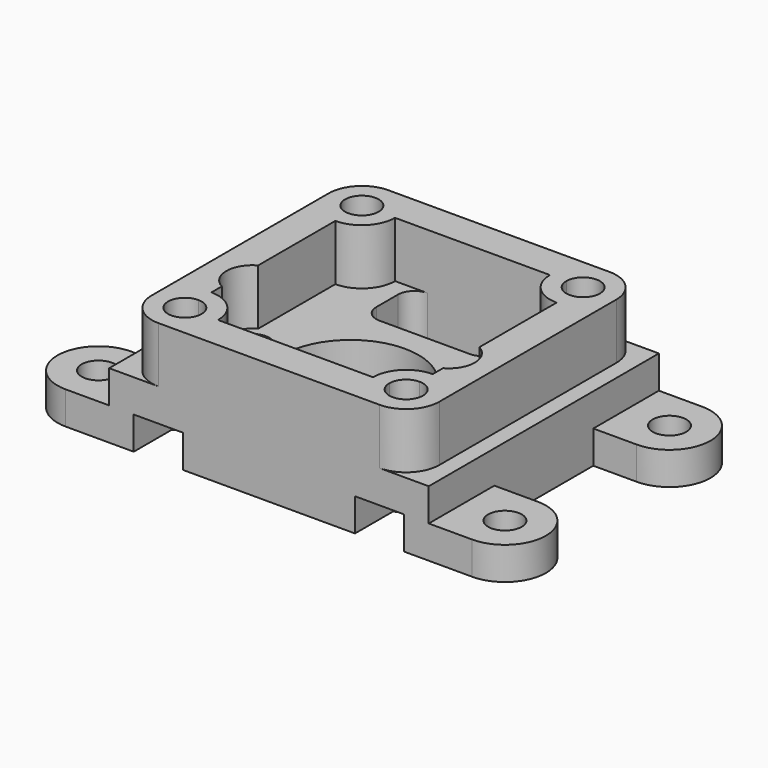
from build123d import *

# Parameters (mm, degrees)
F0_R     = 8.3
F1_DEPTH = 14.8
F0_R_2   = 2.05
F2_DEPTH = 4
F3_DEPTH = 4
F4_R     = 8.3
F5_DEPTH = 6.8
F6_DEPTH = 8


# Not quite as in the source:
# - a feature names something its author has since deleted; it is built from what else it names


with BuildPart() as f1:
    # F0 (on Top) → F1 (new body)
    with BuildSketch(Plane.XY):
        with BuildLine():
            Line((-16.5, 15.2320508076), (-16.5, 17.55))
            Line((-16.5, 17.55), (-17.55, 17.55))
            Line((-17.55, 17.55), (-19.5, 17.55))
            Line((-19.5, 17.55), (-19.5, 7.55))
            Line((-19.5, 7.55), (-19.5, -7.55))
            Line((-19.5, -7.55), (-19.5, -17.55))
            Line((-19.5, -17.55), (-17.55, -17.55))
            Line((-17.55, -17.55), (-16.5, -17.55))
            Line((-16.5, -17.55), (-16.5, -15.2320508076))
            Line((-16.5, -15.2320508076), (-16.5, -11.7679491924))
            Line((-16.5, -11.7679491924), (-13.5, -10.0358983849))
            Line((-13.5, -10.0358983849), (-13.5, -7.8699277969))
            ThreePointArc((-13.5, -7.8699277969), (-15.15, -5.1), (-13.5, -2.3300722031))
            Line((-13.5, -2.3300722031), (-13.5, 10.0358983849))
            Line((-13.5, 10.0358983849), (-16.5, 11.7679491924))
            Line((-16.5, 11.7679491924), (-16.5, 15.2320508076))
        make_face()
        with BuildLine():
            Line((10.5, 11.7679491924), (10.5, 13.5))
            Line((10.5, 13.5), (5.5, 13.5))
            ThreePointArc((5.5, 13.5), (6.9142135624, 12.9142135624), (7.5, 11.5))
            Line((7.5, 11.5), (7.5, 8.2))
            ThreePointArc((7.5, 8.2), (6.9142135624, 6.7857864376), (5.5, 6.2))
            Line((5.5, 6.2), (-5.5, 6.2))
            ThreePointArc((-5.5, 6.2), (-6.9142135624, 6.7857864376), (-7.5, 8.2))
            Line((-7.5, 8.2), (-7.5, 11.5))
            ThreePointArc((-7.5, 11.5), (-6.9142135624, 12.9142135624), (-5.5, 13.5))
            Line((-5.5, 13.5), (-10.5, 13.5))
            Line((-10.5, 13.5), (-10.5, 11.7679491924))
            Line((-10.5, 11.7679491924), (-13.5, 10.0358983849))
            Line((-13.5, 10.0358983849), (-13.5, -2.3300722031))
            ThreePointArc((-13.5, -2.3300722031), (-10.3879361055, -2.3937572171), (-8.85, -5.1))
            ThreePointArc((-8.85, -5.1), (-10.3879361055, -7.8062427829), (-13.5, -7.8699277969))
            Line((-13.5, -7.8699277969), (-13.5, -10.0358983849))
            Line((-13.5, -10.0358983849), (-10.5, -11.7679491924))
            Line((-10.5, -11.7679491924), (-10.5, -13.5))
            Line((-10.5, -13.5), (10.5, -13.5))
            Line((10.5, -13.5), (10.5, -11.7679491924))
            Line((10.5, -11.7679491924), (13.5, -10.0358983849))
            Line((13.5, -10.0358983849), (13.5, -7.8699277969))
            ThreePointArc((13.5, -7.8699277969), (8.85, -5.1), (13.5, -2.3300722031))
            Line((13.5, -2.3300722031), (13.5, 10.0358983849))
            Line((13.5, 10.0358983849), (10.5, 11.7679491924))
        make_face()
        with Locations((0, -5.1)):
            Circle(F0_R, mode=Mode.SUBTRACT)
        Polygon((10.5, 15.2320508076), (10.5, 17.55), (-10.5, 17.55), (-10.5, 15.2320508076), (-10.5, 13.5), (-5.5, 13.5), (5.5, 13.5), (10.5, 13.5), align=None)
        with BuildLine():
            Line((19.5, 17.55), (17.55, 17.55))
            Line((17.55, 17.55), (16.5, 17.55))
            Line((16.5, 17.55), (16.5, 15.2320508076))
            Line((16.5, 15.2320508076), (16.5, 11.7679491924))
            Line((16.5, 11.7679491924), (13.5, 10.0358983849))
            Line((13.5, 10.0358983849), (13.5, -2.3300722031))
            ThreePointArc((13.5, -2.3300722031), (14.7062427829, -3.4879361055), (15.15, -5.1))
            ThreePointArc((15.15, -5.1), (14.7062427829, -6.7120638945), (13.5, -7.8699277969))
            Line((13.5, -7.8699277969), (13.5, -10.0358983849))
            Line((13.5, -10.0358983849), (16.5, -11.7679491924))
            Line((16.5, -11.7679491924), (16.5, -15.2320508076))
            Line((16.5, -15.2320508076), (16.5, -17.55))
            Line((16.5, -17.55), (17.55, -17.55))
            Line((17.55, -17.55), (19.5, -17.55))
            Line((19.5, -17.55), (19.5, -7.55))
            Line((19.5, -7.55), (19.5, 7.55))
            Line((19.5, 7.55), (19.5, 17.55))
        make_face()
        Polygon((-10.5, -17.55), (10.5, -17.55), (10.5, -15.2320508076), (10.5, -13.5), (-10.5, -13.5), (-10.5, -15.2320508076), align=None)
        Polygon((-10.5, 15.2320508076), (-10.5, 17.55), (-16.5, 17.55), (-16.5, 15.2320508076), (-13.5, 16.9641016151), align=None)
        with BuildLine():
            Line((-10.5, 13.5), (-10.5, 15.2320508076))
            Line((-10.5, 15.2320508076), (-13.5, 16.9641016151))
            Line((-13.5, 16.9641016151), (-16.5, 15.2320508076))
            Line((-16.5, 15.2320508076), (-16.5, 11.7679491924))
            Line((-16.5, 11.7679491924), (-13.5, 10.0358983849))
            Line((-13.5, 10.0358983849), (-13.5, 11.45))
            ThreePointArc((-13.5, 11.45), (-14.9495689014, 14.9495689014), (-11.45, 13.5))
            Line((-11.45, 13.5), (-10.5, 13.5))
        make_face()
        Polygon((16.5, 15.2320508076), (16.5, 17.55), (10.5, 17.55), (10.5, 15.2320508076), (13.5, 16.9641016151), align=None)
        with BuildLine():
            Line((16.5, 11.7679491924), (16.5, 15.2320508076))
            Line((16.5, 15.2320508076), (13.5, 16.9641016151))
            Line((13.5, 16.9641016151), (10.5, 15.2320508076))
            Line((10.5, 15.2320508076), (10.5, 13.5))
            Line((10.5, 13.5), (11.45, 13.5))
            ThreePointArc((11.45, 13.5), (13.5, 15.55), (15.55, 13.5))
            ThreePointArc((15.55, 13.5), (14.9495689014, 12.0504310986), (13.5, 11.45))
            Line((13.5, 11.45), (13.5, 10.0358983849))
            Line((13.5, 10.0358983849), (16.5, 11.7679491924))
        make_face()
        with BuildLine():
            Line((11.45, 13.5), (10.5, 13.5))
            Line((10.5, 13.5), (10.5, 11.7679491924))
            Line((10.5, 11.7679491924), (13.5, 10.0358983849))
            Line((13.5, 10.0358983849), (13.5, 11.45))
            ThreePointArc((13.5, 11.45), (12.0504310986, 12.0504310986), (11.45, 13.5))
        make_face()
        with BuildLine():
            Line((-10.5, 11.7679491924), (-10.5, 13.5))
            Line((-10.5, 13.5), (-11.45, 13.5))
            ThreePointArc((-11.45, 13.5), (-12.0504310986, 12.0504310986), (-13.5, 11.45))
            Line((-13.5, 11.45), (-13.5, 10.0358983849))
            Line((-13.5, 10.0358983849), (-10.5, 11.7679491924))
        make_face()
        with BuildLine():
            Line((-10.5, -11.7679491924), (-13.5, -10.0358983849))
            Line((-13.5, -10.0358983849), (-13.5, -11.45))
            ThreePointArc((-13.5, -11.45), (-12.0504310986, -12.0504310986), (-11.45, -13.5))
            Line((-11.45, -13.5), (-10.5, -13.5))
            Line((-10.5, -13.5), (-10.5, -11.7679491924))
        make_face()
        with BuildLine():
            Line((-13.5, -16.9641016151), (-10.5, -15.2320508076))
            Line((-10.5, -15.2320508076), (-10.5, -13.5))
            Line((-10.5, -13.5), (-11.45, -13.5))
            ThreePointArc((-11.45, -13.5), (-14.9495689014, -14.9495689014), (-13.5, -11.45))
            Line((-13.5, -11.45), (-13.5, -10.0358983849))
            Line((-13.5, -10.0358983849), (-16.5, -11.7679491924))
            Line((-16.5, -11.7679491924), (-16.5, -15.2320508076))
            Line((-16.5, -15.2320508076), (-13.5, -16.9641016151))
        make_face()
        Polygon((-16.5, -17.55), (-10.5, -17.55), (-10.5, -15.2320508076), (-13.5, -16.9641016151), (-16.5, -15.2320508076), align=None)
        Polygon((10.5, -17.55), (16.5, -17.55), (16.5, -15.2320508076), (13.5, -16.9641016151), (10.5, -15.2320508076), align=None)
        with BuildLine():
            Line((16.5, -11.7679491924), (13.5, -10.0358983849))
            Line((13.5, -10.0358983849), (13.5, -11.45))
            ThreePointArc((13.5, -11.45), (14.9495689014, -12.0504310986), (15.55, -13.5))
            ThreePointArc((15.55, -13.5), (13.5, -15.55), (11.45, -13.5))
            Line((11.45, -13.5), (10.5, -13.5))
            Line((10.5, -13.5), (10.5, -15.2320508076))
            Line((10.5, -15.2320508076), (13.5, -16.9641016151))
            Line((13.5, -16.9641016151), (16.5, -15.2320508076))
            Line((16.5, -15.2320508076), (16.5, -11.7679491924))
        make_face()
        with BuildLine():
            Line((13.5, -11.45), (13.5, -10.0358983849))
            Line((13.5, -10.0358983849), (10.5, -11.7679491924))
            Line((10.5, -11.7679491924), (10.5, -13.5))
            Line((10.5, -13.5), (11.45, -13.5))
            ThreePointArc((11.45, -13.5), (12.0504310986, -12.0504310986), (13.5, -11.45))
        make_face()
    extrude(amount=F1_DEPTH)

    # F0 (on Top) → F2 (join)
    with BuildSketch(Plane.XY):
        with BuildLine():
            Line((-19.5, 7.55), (-19.5, 17.55))
            Line((-19.5, 17.55), (-24.8, 17.55))
            ThreePointArc((-24.8, 17.55), (-29.8, 12.55), (-24.8, 7.55))
            Line((-24.8, 7.55), (-19.5, 7.55))
        make_face()
        with Locations((-24.8, 12.55)):
            Circle(F0_R_2, mode=Mode.SUBTRACT)
        with BuildLine():
            Line((-19.5, -17.55), (-19.5, -7.55))
            Line((-19.5, -7.55), (-24.8, -7.55))
            ThreePointArc((-24.8, -7.55), (-29.8, -12.55), (-24.8, -17.55))
            Line((-24.8, -17.55), (-19.5, -17.55))
        make_face()
        with Locations((-24.8, -12.55)):
            Circle(F0_R_2, mode=Mode.SUBTRACT)
        with BuildLine():
            Line((24.8, -7.55), (19.5, -7.55))
            Line((19.5, -7.55), (19.5, -17.55))
            Line((19.5, -17.55), (24.8, -17.55))
            ThreePointArc((24.8, -17.55), (29.8, -12.55), (24.8, -7.55))
        make_face()
        with Locations((24.8, -12.55)):
            Circle(F0_R_2, mode=Mode.SUBTRACT)
        with BuildLine():
            Line((24.8, 17.55), (19.5, 17.55))
            Line((19.5, 17.55), (19.5, 7.55))
            Line((19.5, 7.55), (24.8, 7.55))
            ThreePointArc((24.8, 7.55), (29.8, 12.55), (24.8, 17.55))
        make_face()
        with Locations((24.8, 12.55)):
            Circle(F0_R_2, mode=Mode.SUBTRACT)
    extrude(amount=F2_DEPTH)

    # F0 (on Top) → F3 (cut)
    with BuildSketch(Plane.XY):
        with BuildLine():
            Line((16.5, 11.7679491924), (16.5, 15.2320508076))
            Line((16.5, 15.2320508076), (13.5, 16.9641016151))
            Line((13.5, 16.9641016151), (10.5, 15.2320508076))
            Line((10.5, 15.2320508076), (10.5, 13.5))
            Line((10.5, 13.5), (11.45, 13.5))
            ThreePointArc((11.45, 13.5), (13.5, 15.55), (15.55, 13.5))
            ThreePointArc((15.55, 13.5), (14.9495689014, 12.0504310986), (13.5, 11.45))
            Line((13.5, 11.45), (13.5, 10.0358983849))
            Line((13.5, 10.0358983849), (16.5, 11.7679491924))
        make_face()
        with BuildLine():
            Line((11.45, 13.5), (10.5, 13.5))
            Line((10.5, 13.5), (10.5, 11.7679491924))
            Line((10.5, 11.7679491924), (13.5, 10.0358983849))
            Line((13.5, 10.0358983849), (13.5, 11.45))
            ThreePointArc((13.5, 11.45), (12.0504310986, 12.0504310986), (11.45, 13.5))
        make_face()
        Polygon((16.5, 15.2320508076), (16.5, 17.55), (10.5, 17.55), (10.5, 15.2320508076), (13.5, 16.9641016151), align=None)
        with BuildLine():
            Line((-10.5, 13.5), (-10.5, 15.2320508076))
            Line((-10.5, 15.2320508076), (-13.5, 16.9641016151))
            Line((-13.5, 16.9641016151), (-16.5, 15.2320508076))
            Line((-16.5, 15.2320508076), (-16.5, 11.7679491924))
            Line((-16.5, 11.7679491924), (-13.5, 10.0358983849))
            Line((-13.5, 10.0358983849), (-13.5, 11.45))
            ThreePointArc((-13.5, 11.45), (-14.9495689014, 14.9495689014), (-11.45, 13.5))
            Line((-11.45, 13.5), (-10.5, 13.5))
        make_face()
        with BuildLine():
            Line((-10.5, 11.7679491924), (-10.5, 13.5))
            Line((-10.5, 13.5), (-11.45, 13.5))
            ThreePointArc((-11.45, 13.5), (-12.0504310986, 12.0504310986), (-13.5, 11.45))
            Line((-13.5, 11.45), (-13.5, 10.0358983849))
            Line((-13.5, 10.0358983849), (-10.5, 11.7679491924))
        make_face()
        Polygon((-10.5, 15.2320508076), (-10.5, 17.55), (-16.5, 17.55), (-16.5, 15.2320508076), (-13.5, 16.9641016151), align=None)
        with BuildLine():
            Line((13.5, -11.45), (13.5, -10.0358983849))
            Line((13.5, -10.0358983849), (10.5, -11.7679491924))
            Line((10.5, -11.7679491924), (10.5, -13.5))
            Line((10.5, -13.5), (11.45, -13.5))
            ThreePointArc((11.45, -13.5), (12.0504310986, -12.0504310986), (13.5, -11.45))
        make_face()
        with BuildLine():
            Line((16.5, -11.7679491924), (13.5, -10.0358983849))
            Line((13.5, -10.0358983849), (13.5, -11.45))
            ThreePointArc((13.5, -11.45), (14.9495689014, -12.0504310986), (15.55, -13.5))
            ThreePointArc((15.55, -13.5), (13.5, -15.55), (11.45, -13.5))
            Line((11.45, -13.5), (10.5, -13.5))
            Line((10.5, -13.5), (10.5, -15.2320508076))
            Line((10.5, -15.2320508076), (13.5, -16.9641016151))
            Line((13.5, -16.9641016151), (16.5, -15.2320508076))
            Line((16.5, -15.2320508076), (16.5, -11.7679491924))
        make_face()
        Polygon((10.5, -17.55), (16.5, -17.55), (16.5, -15.2320508076), (13.5, -16.9641016151), (10.5, -15.2320508076), align=None)
        with BuildLine():
            Line((-13.5, -16.9641016151), (-10.5, -15.2320508076))
            Line((-10.5, -15.2320508076), (-10.5, -13.5))
            Line((-10.5, -13.5), (-11.45, -13.5))
            ThreePointArc((-11.45, -13.5), (-14.9495689014, -14.9495689014), (-13.5, -11.45))
            Line((-13.5, -11.45), (-13.5, -10.0358983849))
            Line((-13.5, -10.0358983849), (-16.5, -11.7679491924))
            Line((-16.5, -11.7679491924), (-16.5, -15.2320508076))
            Line((-16.5, -15.2320508076), (-13.5, -16.9641016151))
        make_face()
        with BuildLine():
            Line((-10.5, -11.7679491924), (-13.5, -10.0358983849))
            Line((-13.5, -10.0358983849), (-13.5, -11.45))
            ThreePointArc((-13.5, -11.45), (-12.0504310986, -12.0504310986), (-11.45, -13.5))
            Line((-11.45, -13.5), (-10.5, -13.5))
            Line((-10.5, -13.5), (-10.5, -11.7679491924))
        make_face()
        Polygon((-16.5, -17.55), (-10.5, -17.55), (-10.5, -15.2320508076), (-13.5, -16.9641016151), (-16.5, -15.2320508076), align=None)
    extrude(amount=F3_DEPTH, mode=Mode.SUBTRACT)

    # F4 (on face) → F5 (cut)
    with BuildSketch(Plane.XY.offset(14.8)):
        with BuildLine():
            ThreePointArc((13.5, 9.45), (10.6362175362, 10.6362175362), (9.45, 13.5))
            Line((9.45, 13.5), (5.5, 13.5))
            ThreePointArc((5.5, 13.5), (6.9142135624, 12.9142135624), (7.5, 11.5))
            Line((7.5, 11.5), (7.5, 8.2))
            ThreePointArc((7.5, 8.2), (6.9142135624, 6.7857864376), (5.5, 6.2))
            Line((5.5, 6.2), (-5.5, 6.2))
            ThreePointArc((-5.5, 6.2), (-6.9142135624, 6.7857864376), (-7.5, 8.2))
            Line((-7.5, 8.2), (-7.5, 11.5))
            ThreePointArc((-7.5, 11.5), (-6.9142135624, 12.9142135624), (-5.5, 13.5))
            Line((-5.5, 13.5), (-9.45, 13.5))
            ThreePointArc((-9.45, 13.5), (-10.6362175362, 10.6362175362), (-13.5, 9.45))
            Line((-13.5, 9.45), (-13.5, -2.3300722031))
            ThreePointArc((-13.5, -2.3300722031), (-10.3879361055, -2.3937572171), (-8.85, -5.1))
            ThreePointArc((-8.85, -5.1), (-10.3879361055, -7.8062427829), (-13.5, -7.8699277969))
            Line((-13.5, -7.8699277969), (-13.5, -9.45))
            ThreePointArc((-13.5, -9.45), (-10.6362175362, -10.6362175362), (-9.45, -13.5))
            Line((-9.45, -13.5), (9.45, -13.5))
            ThreePointArc((9.45, -13.5), (10.6362175362, -10.6362175362), (13.5, -9.45))
            Line((13.5, -9.45), (13.5, -7.8699277969))
            ThreePointArc((13.5, -7.8699277969), (8.85, -5.1), (13.5, -2.3300722031))
            Line((13.5, -2.3300722031), (13.5, 9.45))
        make_face()
        with Locations((0, -5.1)):
            Circle(F4_R, mode=Mode.SUBTRACT)
        with BuildLine():
            Line((17.55, 17.55), (13.5, 17.55))
            ThreePointArc((13.5, 17.55), (16.3637824638, 16.3637824638), (17.55, 13.5))
            Line((17.55, 13.5), (17.55, 17.55))
        make_face()
        Polygon((17.55, 17.55), (17.55, 13.5), (17.55, -13.5), (17.55, -17.55), (19.5, -17.55), (19.5, 17.55), align=None)
        with BuildLine():
            ThreePointArc((-17.55, 13.5), (-16.3637824658, 16.3637824618), (-13.5000000055, 17.55))
            Line((-13.5000000055, 17.55), (-17.55, 17.55))
            Line((-17.55, 17.55), (-17.55, 13.5))
        make_face()
        with BuildLine():
            Line((17.55, -17.55), (17.55, -13.5))
            ThreePointArc((17.55, -13.5), (16.3637824652, -16.3637824624), (13.500000004, -17.55))
            Line((13.500000004, -17.55), (17.55, -17.55))
        make_face()
        Polygon((-17.55, 13.5), (-17.55, 17.55), (-19.5, 17.55), (-19.5, -17.55), (-17.55, -17.55), (-17.55, -13.5), align=None)
        with BuildLine():
            ThreePointArc((-13.5, -17.55), (-16.3637824638, -16.3637824638), (-17.55, -13.5))
            Line((-17.55, -13.5), (-17.55, -17.55))
            Line((-17.55, -17.55), (-13.5, -17.55))
        make_face()
    extrude(amount=-F5_DEPTH, mode=Mode.SUBTRACT)

    # F0 (on Top) → F6 (join)
    with BuildSketch(Plane.XY):
        with BuildLine():
            ThreePointArc((-8.85, -5.1), (-10.3879361055, -2.3937572171), (-13.5, -2.3300722031))
            Line((-13.5, -2.3300722031), (-13.5, -3.7026811388))
            ThreePointArc((-13.5, -3.7026811388), (-11.2491671291, -3.1924492143), (-9.95, -5.1))
            ThreePointArc((-9.95, -5.1), (-11.2491671291, -7.0075507857), (-13.5, -6.4973188612))
            Line((-13.5, -6.4973188612), (-13.5, -7.8699277969))
            ThreePointArc((-13.5, -7.8699277969), (-10.3879361055, -7.8062427829), (-8.85, -5.1))
        make_face()
        with BuildLine():
            Line((-13.5, -3.7026811388), (-13.5, -2.3300722031))
            ThreePointArc((-13.5, -2.3300722031), (-15.15, -5.1), (-13.5, -7.8699277969))
            Line((-13.5, -7.8699277969), (-13.5, -6.4973188612))
            ThreePointArc((-13.5, -6.4973188612), (-14.05, -5.1), (-13.5, -3.7026811388))
        make_face()
        with BuildLine():
            Line((13.5, -3.7026811388), (13.5, -2.3300722031))
            ThreePointArc((13.5, -2.3300722031), (8.85, -5.1), (13.5, -7.8699277969))
            Line((13.5, -7.8699277969), (13.5, -6.4973188612))
            ThreePointArc((13.5, -6.4973188612), (9.95, -5.1), (13.5, -3.7026811388))
        make_face()
        with BuildLine():
            ThreePointArc((15.15, -5.1), (14.7062427829, -3.4879361055), (13.5, -2.3300722031))
            Line((13.5, -2.3300722031), (13.5, -3.7026811388))
            ThreePointArc((13.5, -3.7026811388), (13.9075507857, -4.3491671291), (14.05, -5.1))
            ThreePointArc((14.05, -5.1), (13.9075507857, -5.8508328709), (13.5, -6.4973188612))
            Line((13.5, -6.4973188612), (13.5, -7.8699277969))
            ThreePointArc((13.5, -7.8699277969), (14.7062427829, -6.7120638945), (15.15, -5.1))
        make_face()
    extrude(amount=F6_DEPTH)


solid = f1.part
